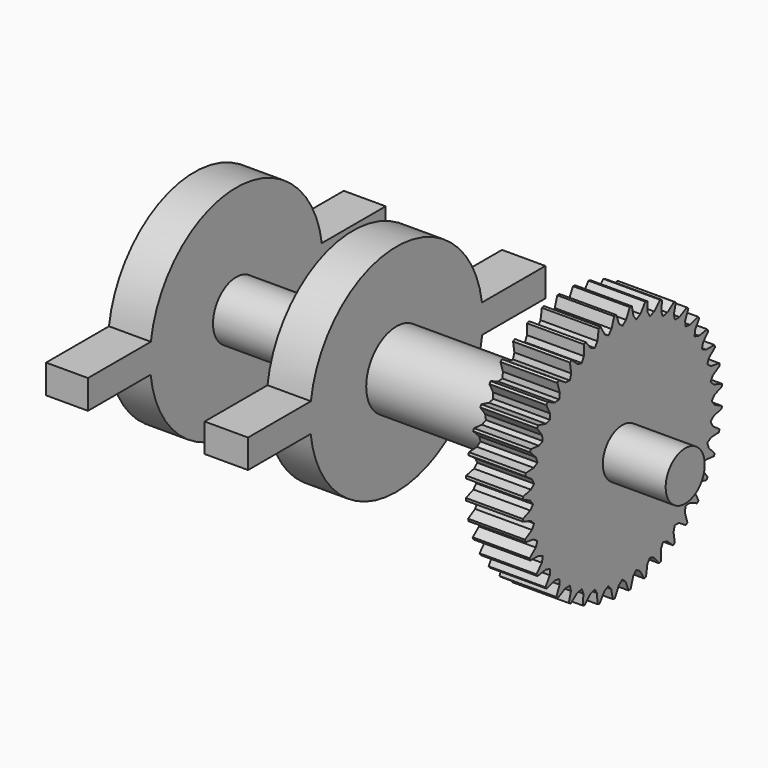
from build123d import *

# Parameters (mm, degrees)
F1_DEPTH  = 5.08
F5_R      = 4.1520133517
F6_DEPTH  = 26.924
F7_R      = 4.1520133517
F8_DEPTH  = 6.35
F9_R      = 4.1476855986
F10_DEPTH = 25.4
F11_W     = 84.2210557312
F11_H     = 11.4299990237
F11_W_2   = 84.8226295784
F11_H_2   = 20.7544751465
F12_DEPTH = 13.208
F13_R     = 21.1650894072
F13_R_2   = 4.1476855986
F14_DEPTH = 9.652
F16_DEPTH = 25.4
F17_COUNT = 40
F18_R     = 6.4114387171
F19_DEPTH = 28.702
F20_R     = 6.4114387171
F21_DEPTH = 6.604
F22_DEPTH = 7.366
F23_R     = 4.9462001283
F24_DEPTH = 19.812
F25_R     = 4.9462001283
F26_DEPTH = 7.112
F27_R     = 3.6385680332
F27_R_2   = 2.2751870905
F28_DEPTH = 7.62
F29_DEPTH = 9.144
F30_R     = 39.4862811726
F30_R_2   = 3.6385680332
F30_R_3   = 2.2751870905
F31_DEPTH = 69.342


# Not quite as in the source:
# - a feature of the source that left no trace in its solid (it failed there, or was rolled back) is left out
# - a feature names something its author has since deleted; it is built from what else it names


with BuildPart() as f1:
    # F0 (on Right) → F1 (new body)
    with BuildSketch(Plane.YZ):
        with BuildLine():
            Line((0, -32.8725613654), (0, -20.4708488309))
            ThreePointArc((0, -20.4708488309), (-2.2257968393, -20.3494835386), (-4.425201565, -19.9868267358))
            Line((-4.425201565, -19.9868267358), (-4.425201565, -32.8138524732))
            Line((-4.425201565, -32.8138524732), (0, -32.8725613654))
        make_face()
    extrude(amount=F1_DEPTH)


with BuildPart() as f1b:
    # F0 (on Right) → F1, piece 2 (new body)
    with BuildSketch(Plane.YZ):
        with BuildLine():
            ThreePointArc((-4.425201565, 19.9868267358), (-2.2257968393, 20.3494835386), (0, 20.4708488309))
            Line((0, 20.4708488309), (0, 32.8725613654))
            Line((0, 32.8725613654), (-4.425201565, 32.8138524732))
            Line((-4.425201565, 32.8138524732), (-4.425201565, 19.9868267358))
        make_face()
    extrude(amount=F1_DEPTH)


with BuildPart() as f6:
    # F5 (on face) → F6 (new body)
    with BuildSketch(Plane(origin=(0, 0, 0), x_dir=(0, -1, 0), z_dir=(-1, 0, 0))):
        Circle(F5_R)
    extrude(amount=F6_DEPTH)

    # F7 (on face) → F8 (join)
    with BuildSketch(Plane(origin=(-26.924, 0, 0), x_dir=(0, -1, 0), z_dir=(-1, 0, 0))):
        with BuildLine():
            ThreePointArc((4.7857561149, -17.3808329088), (14.3400285329, -10.9252183442), (18.0276680187, 0))
            ThreePointArc((18.0276680187, 0), (14.1380676404, 11.1853411923), (4.1476855986, 17.5440450971))
            ThreePointArc((4.1476855986, 17.5440450971), (2.0878928945, 17.9063541084), (0, 18.0276680187))
            ThreePointArc((0, 18.0276680187), (-18.0276680187, 0), (0, -18.0276680187))
            ThreePointArc((0, -18.0276680187), (2.4146354409, -17.8652273952), (4.7857561149, -17.3808329088))
        make_face()
        Circle(F7_R, mode=Mode.SUBTRACT)
        with BuildLine():
            ThreePointArc((0, 18.0276680187), (2.0878928945, 17.9063541084), (4.1476855986, 17.5440450971))
            Line((4.1476855986, 17.5440450971), (4.1476855986, 42.3946790397))
            Line((4.1476855986, 42.3946790397), (0, 39.4170172513))
            Line((0, 39.4170172513), (0, 18.0276680187))
        make_face()
        with BuildLine():
            Line((4.7857561149, -37.1514819562), (4.7857561149, -17.3808329088))
            ThreePointArc((4.7857561149, -17.3808329088), (2.4146354409, -17.8652273952), (0, -18.0276680187))
            Line((0, -18.0276680187), (0, -39.4910760224))
            Line((0, -39.4910760224), (4.7857561149, -37.1514819562))
        make_face()
    extrude(amount=-F8_DEPTH)

    # F9 (on face) → F10 (join)
    with BuildSketch(Plane(origin=(-26.924, 0, 0), x_dir=(0, -1, 0), z_dir=(-1, 0, 0))):
        Circle(F9_R)
    extrude(amount=F10_DEPTH)


with BuildPart() as f12_tool:
    # F11 (on Front) → F12 (new body)
    with BuildSketch(Plane.XZ):
        with Locations((-29.9285547808, 38.2002647966)):
            Rectangle(F11_W, F11_H)
        with Locations((-28.1238160096, -43.1632902473)):
            Rectangle(F11_W_2, F11_H_2)
    extrude(amount=F12_DEPTH)


with BuildPart() as f1_1:
    add(f1.part)

    # F12: cut by f12_tool
    add(f12_tool.part, mode=Mode.SUBTRACT)


with BuildPart() as f1b_1:
    add(f1b.part)

    # F12: cut by f12_tool
    add(f12_tool.part, mode=Mode.SUBTRACT)


with BuildPart() as f6_1:
    add(f6.part)

    # F12: cut by f12_tool
    add(f12_tool.part, mode=Mode.SUBTRACT)

    # F13 (on face) → F14 (join)
    with BuildSketch(Plane(origin=(-52.324, 0, 0), x_dir=(0, -1, 0), z_dir=(-1, 0, 0))):
        Circle(F13_R)
        Circle(F13_R_2, mode=Mode.SUBTRACT)
        Circle(F13_R_2)
    extrude(amount=F14_DEPTH)

    # F15 (on face) → F16 (cut)
    with BuildSketch(Plane(origin=(-61.976, 0, 0), x_dir=(0, -1, 0), z_dir=(-1, 0, 0))):
        with BuildLine():
            ThreePointArc((1.310742254, 21.1244636466), (-0.1339755114, 21.1646653689), (-1.5780685539, 21.1061770402))
            Line((-1.5780685539, 21.1061770402), (-0.7766649942, 19.5370744914))
            Line((-0.7766649942, 19.5370744914), (0, 18.9521759748))
            Line((0, 18.9521759748), (0.6955460995, 19.5370744914))
            Line((0.6955460995, 19.5370744914), (1.310742254, 21.1244636466))
        make_face()
    f16 = extrude(amount=-F16_DEPTH, mode=Mode.SUBTRACT)

    # F17: F16 ×40 about axis
    f17_axis = Axis((-52.324, 0, 0), (1, 0, 0))
    for i in range(1, F17_COUNT):
        add(f16.rotate(f17_axis, i * 360 / F17_COUNT), mode=Mode.SUBTRACT)

    # F18 (on face) → F19 (join)
    with BuildSketch(Plane(origin=(-61.976, 0, 0), x_dir=(0, -1, 0), z_dir=(-1, 0, 0))):
        Circle(F18_R)
    extrude(amount=F19_DEPTH)

    # F20 (on face) → F21 (join)
    with BuildSketch(Plane(origin=(-90.678, 0, 0), x_dir=(0, -1, 0), z_dir=(-1, 0, 0))):
        with BuildLine():
            ThreePointArc((18.1928136018, -2.2680452093), (18.2984023965, -1.1362066518), (18.3336438228, 0))
            ThreePointArc((18.3336438228, 0), (18.2874517996, 1.3006162002), (18.1491084935, 2.5946785375))
            ThreePointArc((18.1491084935, 2.5946785375), (0, 18.3336438228), (-18.1491084935, 2.5946785375))
            ThreePointArc((-18.1491084935, 2.5946785375), (-18.3329033695, 0.1647721666), (-18.1928136018, -2.2680452093))
            ThreePointArc((-18.1928136018, -2.2680452093), (0, -18.3336438228), (18.1928136018, -2.2680452093))
        make_face()
        Circle(F20_R, mode=Mode.SUBTRACT)
        Circle(F20_R)
    extrude(amount=F21_DEPTH)

    # F20 (on face) → F22 (join)
    with BuildSketch(Plane(origin=(-90.678, 0, 0), x_dir=(0, -1, 0), z_dir=(-1, 0, 0))):
        with BuildLine():
            ThreePointArc((18.1928136018, -2.2680452093), (18.2984023965, -1.1362066518), (18.3336438228, 0))
            ThreePointArc((18.3336438228, 0), (18.2874517996, 1.3006162002), (18.1491084935, 2.5946785375))
            ThreePointArc((18.1491084935, 2.5946785375), (0, 18.3336438228), (-18.1491084935, 2.5946785375))
            ThreePointArc((-18.1491084935, 2.5946785375), (-18.3329033695, 0.1647721666), (-18.1928136018, -2.2680452093))
            ThreePointArc((-18.1928136018, -2.2680452093), (0, -18.3336438228), (18.1928136018, -2.2680452093))
        make_face()
        with BuildLine():
            ThreePointArc((18.1491084935, 2.5946785375), (18.2874517996, 1.3006162002), (18.3336438228, 0))
            ThreePointArc((18.3336438228, 0), (18.2984023965, -1.1362066518), (18.1928136018, -2.2680452093))
            Line((18.1928136018, -2.2680452093), (31.4867012203, -2.2680452093))
            Line((31.4867012203, -2.2680452093), (31.4867012203, 0))
            Line((31.4867012203, 0), (31.4867012203, 2.5946785375))
            Line((31.4867012203, 2.5946785375), (18.1491084935, 2.5946785375))
        make_face()
        with BuildLine():
            ThreePointArc((-18.1928136018, -2.2680452093), (-18.3329033695, 0.1647721666), (-18.1491084935, 2.5946785375))
            Line((-18.1491084935, 2.5946785375), (-31.6057130694, 2.5946785375))
            Line((-31.6057130694, 2.5946785375), (-31.6057130694, 0))
            Line((-31.6057130694, 0), (-31.6057130694, -2.2680452093))
            Line((-31.6057130694, -2.2680452093), (-18.1928136018, -2.2680452093))
        make_face()
    extrude(amount=F22_DEPTH)

    # F23 (on face) → F24 (join)
    with BuildSketch(Plane(origin=(-98.044, 0, 0), x_dir=(0, -1, 0), z_dir=(-1, 0, 0))):
        Circle(F23_R)
    extrude(amount=F24_DEPTH)

    # F25 (on face) → F26 (join)
    with BuildSketch(Plane(origin=(-117.856, 0, 0), x_dir=(0, -1, 0), z_dir=(-1, 0, 0))):
        with BuildLine():
            ThreePointArc((18.1856173017, -2.2592737805), (18.2904354514, -1.1317975338), (18.3254193583, 0))
            ThreePointArc((18.3254193583, 0), (18.2775592124, 1.3235648444), (18.1342287653, 2.6402162311))
            ThreePointArc((18.1342287653, 2.6402162311), (-0.0038469595, 18.3254189546), (-18.1353356606, 2.6326023508))
            ThreePointArc((-18.1353356606, 2.6326023508), (-18.3243779894, 0.1953610999), (-18.1873408867, -2.2453565711))
            ThreePointArc((-18.1873408867, -2.2453565711), (-0.0070117663, -18.3254180169), (18.1856173017, -2.2592737805))
        make_face()
        Circle(F25_R, mode=Mode.SUBTRACT)
        Circle(F25_R)
        with BuildLine():
            ThreePointArc((-18.1873408867, -2.2453565711), (-18.3243779894, 0.1953610999), (-18.1353356606, 2.6326023508))
            Line((-18.1353356606, 2.6326023508), (-31.6914805857, 2.6326023508))
            Line((-31.6914805857, 2.6326023508), (-31.6914805857, -2.2453565711))
            Line((-31.6914805857, -2.2453565711), (-18.1873408867, -2.2453565711))
        make_face()
        with BuildLine():
            ThreePointArc((18.1342287653, 2.6402162311), (18.2775592124, 1.3235648444), (18.3254193583, 0))
            ThreePointArc((18.3254193583, 0), (18.2904354514, -1.1317975338), (18.1856173017, -2.2592737805))
            Line((18.1856173017, -2.2592737805), (31.477529748, -2.2592737805))
            Line((31.477529748, -2.2592737805), (31.477529748, 2.6402162311))
            Line((31.477529748, 2.6402162311), (18.1342287653, 2.6402162311))
        make_face()
    extrude(amount=F26_DEPTH)


with BuildPart() as f28:
    # F27 (on face) → F28 (new body)
    with BuildSketch(Plane.YZ.offset(10.922)):
        with Locations((0, 15.5682079494)):
            Circle(F27_R)
        with Locations((0, 15.5682079494)):
            Circle(F27_R_2, mode=Mode.SUBTRACT)
    extrude(amount=F28_DEPTH)

    # F29 (add): a face of the model
    f29_faces = [f28.faces().sort_by_distance(p)[0] for p in [
        (18.542, -3.535653788, 15.5682079494),
    ]]
    extrude(f29_faces, amount=F29_DEPTH)


with BuildPart() as f31_tool:
    # F30 (on face) → F31 (new body)
    with BuildSketch(Plane.YZ.offset(27.686)):
        Circle(F30_R)
        with Locations((0, 15.5682079494)):
            Circle(F30_R_2, mode=Mode.SUBTRACT)
        with Locations((0, 15.5682079494)):
            Circle(F30_R_2)
        with Locations((0, 15.5682079494)):
            Circle(F30_R_3, mode=Mode.SUBTRACT)
        with Locations((0, 15.5682079494)):
            Circle(F30_R_3)
    extrude(amount=-F31_DEPTH)


with BuildPart() as f1_2:
    add(f1_1.part)

    # F31: cut by f31_tool
    add(f31_tool.part, mode=Mode.SUBTRACT)


with BuildPart() as f1b_2:
    add(f1b_1.part)

    # F31: cut by f31_tool
    add(f31_tool.part, mode=Mode.SUBTRACT)


with BuildPart() as f6_2:
    add(f6_1.part)

    # F31: cut by f31_tool
    add(f31_tool.part, mode=Mode.SUBTRACT)


with BuildPart() as f28_1:
    add(f28.part)

    # F31: cut by f31_tool
    add(f31_tool.part, mode=Mode.SUBTRACT)


solid = f6_2.part
